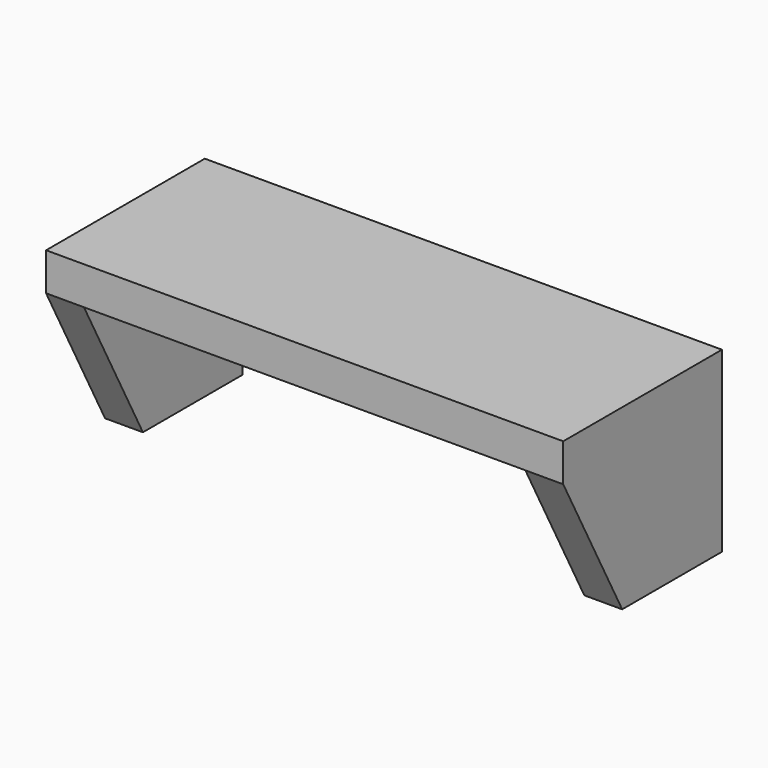
from build123d import *

# Parameters (mm, degrees)
F1_DEPTH     = 16.2
F3_DEPTH     = 10
F4_T4_DEPTH  = 5
F4_T10_DEPTH = 5


# Not quite as in the source:
# - a fillet or chamfer that OpenCascade refuses, or shapes differently, is made with other operations: its cross-section is extruded or revolved along the edge and cut away or added


with BuildPart() as f1:
    # F0 (on Front) → F1 (new body)
    with BuildSketch(Plane.XZ):
        Polygon((-29.15, 0), (0, 0), (29.15, 0), (29.15, -18.5), (34.15, -18.5), (34.15, 5), (0, 5), (-34.15, 5), (-34.15, -18.5), (-29.15, -18.5), align=None)
    extrude(amount=F1_DEPTH)

    # F2 (on face) → F3 (join)
    with BuildSketch(Plane.XZ.offset(16.2)):
        Polygon((34.15, 5), (-34.15, 5), (-34.15, 0), (-29.15, 0), (29.15, 0), (34.15, 0), align=None)
    extrude(amount=F3_DEPTH)

    # F4: chamfer of 10 x 19 on 2 edges, made by hand


with BuildPart() as f4_tool2:
    # F4_s3 → F4_t4 (new body)
    with BuildSketch(Plane.YZ.offset(29.15)):
        Polygon((-26.2, 0), (-16.2, -19), (-16.2, 0), align=None)
    extrude(amount=F4_T4_DEPTH)

    split(bisect_by=Plane.XZ.offset(26.2), keep=Keep.BOTTOM)

    split(bisect_by=Plane.XY.offset(-18.5), keep=Keep.TOP)


with BuildPart() as f1_1:
    add(f1.part)

    # F4_t1: union F4_tool2
    add(f4_tool2.part)


with BuildPart() as f4_tool8:
    # F4_s9 → F4_t10 (new body)
    with BuildSketch(Plane.YZ.offset(-34.15)):
        Polygon((-26.2, 0), (-16.2, -19), (-16.2, 0), align=None)
    extrude(amount=F4_T10_DEPTH)

    split(bisect_by=Plane.XZ.offset(26.2), keep=Keep.BOTTOM)

    split(bisect_by=Plane.XY.offset(-18.5), keep=Keep.TOP)


with BuildPart() as f1_2:
    add(f1_1.part)

    # F4_t7: union F4_tool8
    add(f4_tool8.part)


solid = f1_2.part
